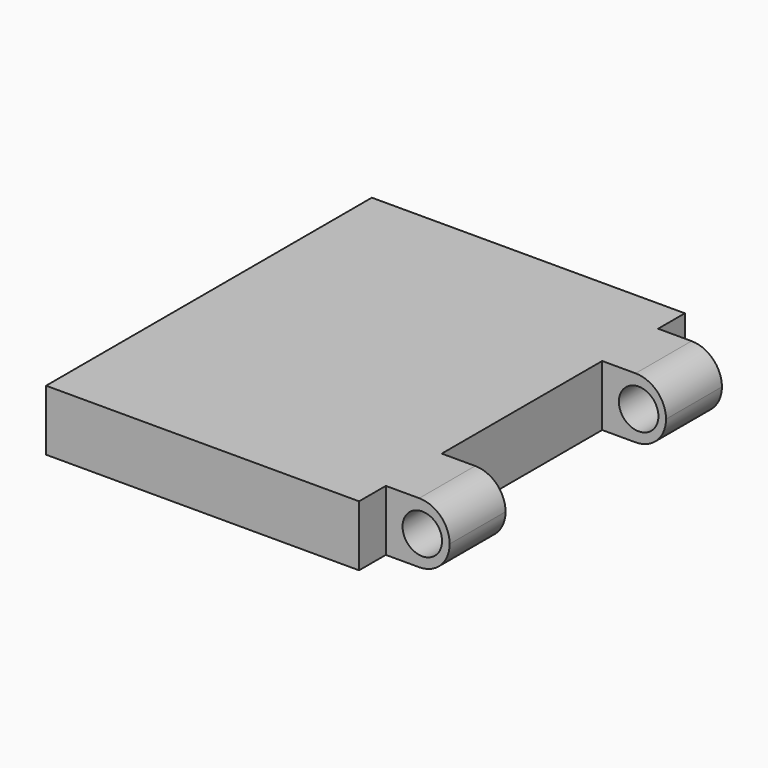
from build123d import *

# Parameters (mm, degrees)
F0_W     = 20.6
F0_H     = 4
F1_DEPTH = 13.4
F2_W     = 4.6
F2_H     = 4
F3_DEPTH = 4.2
F4_R     = 1.3
F5_DEPTH = 25
F6_R     = 1.99999


# Not quite as in the source:
# - a fillet or chamfer is up to 0.001 mm smaller than in the source, because OpenCascade refuses the exact size


with BuildPart() as f1:
    # F0 (on Front) → F1 (new body)
    with BuildSketch(Plane.XZ):
        with Locations((-17.0743378759, 29.5677930117)):
            Rectangle(F0_W, F0_H)
    extrude(amount=F1_DEPTH)

    # F2 (on face) → F3 (join)
    with BuildSketch(Plane.YZ.offset(-6.7743378759)):
        with Locations((-8.9, 29.5677930117)):
            Rectangle(F2_W, F2_H)
    extrude(amount=F3_DEPTH)

    # F4 (on face) → F5 (cut)
    with BuildSketch(Plane.XZ.offset(11.2)):
        with Locations((-4.3743378759, 29.5677930117)):
            Circle(F4_R)
    extrude(amount=-F5_DEPTH, mode=Mode.SUBTRACT)

    # F6 (radius 2 in the source; OpenCascade refuses exactly that, so slightly less here)
    f6_edges = [f1.edges().sort_by_distance(p)[0] for p in [
        (-2.574338, -8.9, 31.567793),
        (-2.574338, -8.9, 27.567793),
    ]]
    fillet(f6_edges, radius=F6_R)

    # F7: F1 across face


with BuildPart() as f1_1:
    add(f1.part)
    add(f1.part.mirror(Plane(origin=(-17.0743378759, 0, 29.5677930117), x_dir=(1, 0, 0), z_dir=(0, 1, 0))))


solid = f1_1.part
